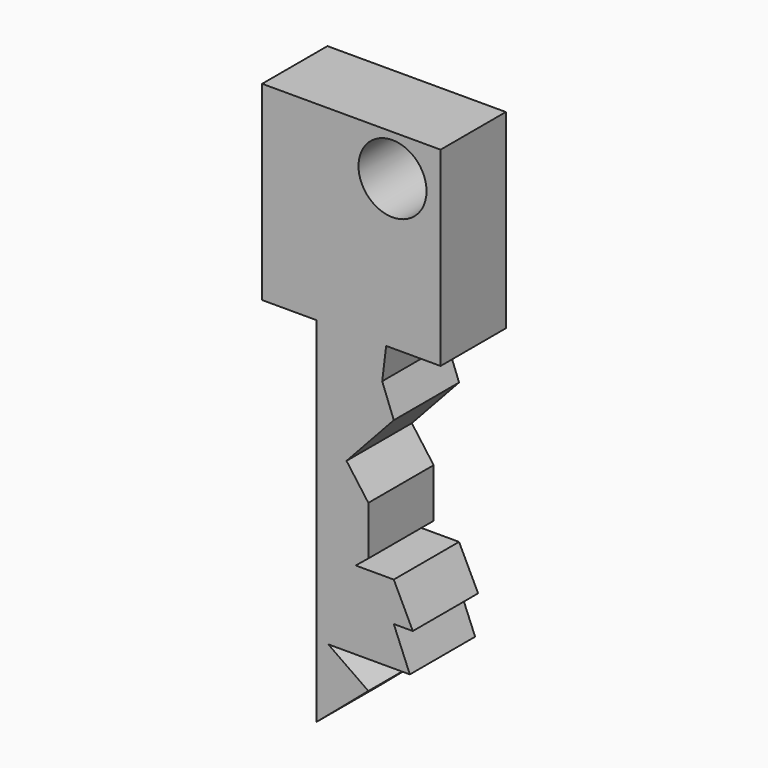
from build123d import *

# Parameters (mm, degrees)
F5_DEPTH = 3.81
F6_R     = 1.5875
F7_DEPTH = 25.4


# Not quite as in the source:
# - a feature of the source that left no trace in its solid (it failed there, or was rolled back) is left out


with BuildPart() as f5:
    # F3 (on offset) → F5 (new body)
    with BuildSketch(Plane.XZ.offset(25.4)):
        Polygon((15.9794489164, 25.4), (7.6507270483, 25.4), (7.6507270483, 16.51), (10.1907270483, 16.51), (10.1907270483, 0), (12.6087698864, 2.0575941857), (10.7351641334, 3.3673260217), (14.5451641334, 3.3673260217), (13.7953708033, 5.1956650805), (14.6843708033, 5.1956650805), (13.7953708033, 7.0228768909), (12.0173708033, 7.0228768909), (12.6087698864, 7.5033882066), (12.6087698864, 9.7893882066), (11.5895427104, 11.1838041431), (13.7953708033, 13.5722395859), (13.2549618376, 14.9972077083), (13.4394489164, 16.51), (15.9794489164, 16.51), align=None)
    extrude(amount=F5_DEPTH)

    # F6 (on face) → F7 (cut)
    with BuildSketch(Plane.XZ.offset(29.21)):
        with Locations((13.7358959764, 23.4795026481)):
            Circle(F6_R)
    extrude(amount=-F7_DEPTH, mode=Mode.SUBTRACT)


solid = f5.part
